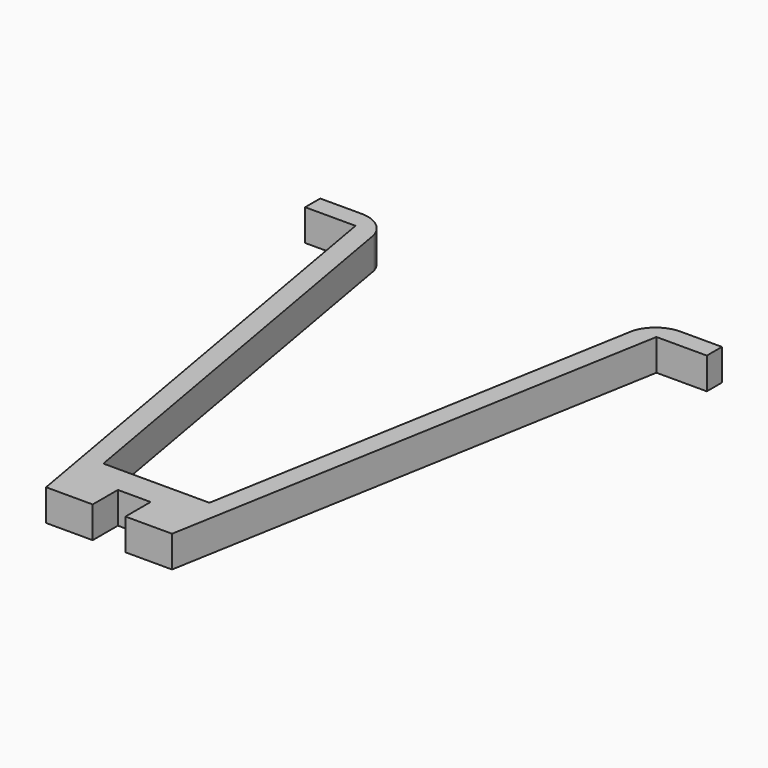
from build123d import *

# Parameters (mm, degrees)
F1_DEPTH    = 5
F2_T1_DEPTH = 28.770290161


# Not quite as in the source:
# - a fillet or chamfer that OpenCascade refuses, or shapes differently, is made with other operations: its cross-section is extruded or revolved along the edge and cut away or added


with BuildPart() as f1:
    # F0 (on Top) → F1 (new body)
    with BuildSketch(Plane.XY):
        Polygon((-10, 0), (-2.6, 0), (-2.6, 5), (0, 5), (2.6, 5), (2.6, 0), (10, 0), (23.8918542134, 78.784620241), (31.8918542134, 78.784620241), (31.8918542134, 81.784620241), (20.5755738699, 81.784620241), (20.5755738699, 78.3334689187), (8.4202014333, 9.3969262079), (3.4202014333, 9.3969262079), (0, 9.3969262079), (-8.4202014333, 9.3969262079), (-20.5755738699, 78.3334689187), (-20.5755738699, 81.784620241), (-31.8918542134, 81.784620241), (-31.8918542134, 78.784620241), (-23.8918542134, 78.784620241), align=None)
    extrude(amount=F1_DEPTH)

    # F2: fillet of radius 5 on 2 edges, made by hand

    # F2_s2 → F2_t1 (cut)
    with BuildSketch(Plane.XY.offset(-11.8851450805)):
        with BuildLine():
            ThreePointArc((-25.3296319021, 81.784620241), (-22.3923068766, 80.8308680948), (-20.5755738699, 78.3334689187))
            Line((-20.5755738699, 78.3334689187), (-20.5755738699, 81.784620241))
            Line((-20.5755738699, 81.784620241), (-25.3296319021, 81.784620241))
        make_face()
        with BuildLine():
            ThreePointArc((20.5755738699, 78.3334689187), (22.3923068766, 80.8308680948), (25.3296319021, 81.784620241))
            Line((25.3296319021, 81.784620241), (20.5755738699, 81.784620241))
            Line((20.5755738699, 81.784620241), (20.5755738699, 78.3334689187))
        make_face()
    extrude(amount=F2_T1_DEPTH, mode=Mode.SUBTRACT)


solid = f1.part
